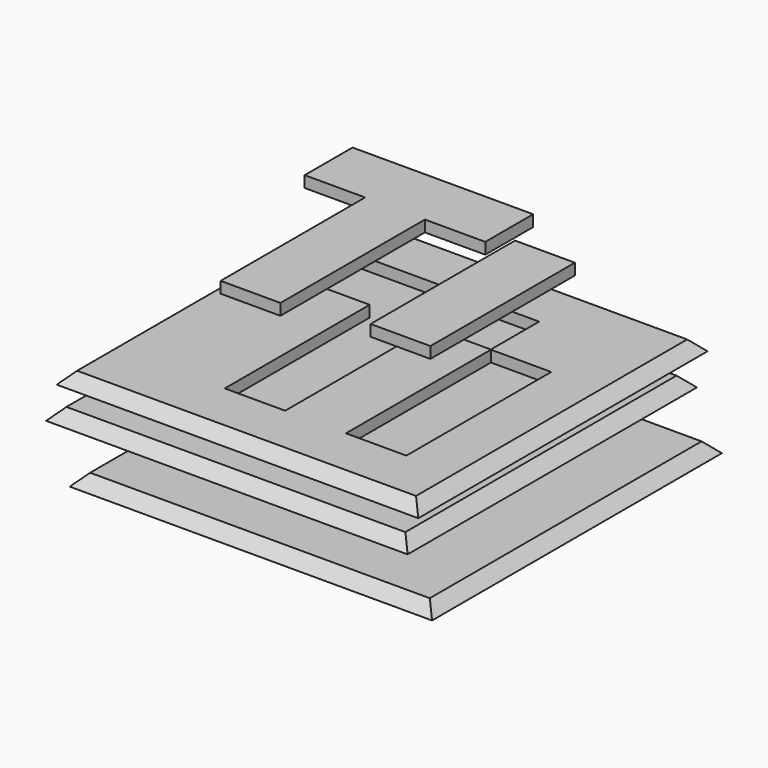
from build123d import *

# Parameters (mm, degrees)
F0_W      = 192
F0_H      = 192
F1_DEPTH  = 6
F2_SIZE   = 5.99999
F4_W      = 191.6
F4_H      = 191.6
F5_DEPTH  = 6
F6_SIZE   = 5.99999
F8_W      = 191.6
F8_H      = 191.6
F9_DEPTH  = 6
F10_SIZE  = 5.99999
F11_W     = 32
F11_H     = 96
F12_DEPTH = 25
F13_W     = 32
F13_H     = 96
F14_DEPTH = 62.001
F16_W     = 31.7
F16_H     = 95.7
F17_DEPTH = 6


# Not quite as in the source:
# - a fillet or chamfer is up to 0.001 mm smaller than in the source, because OpenCascade refuses the exact size


with BuildPart() as f1:
    # F0 (on Top) → F1 (new body)
    with BuildSketch(Plane.XY):
        with Locations((-14.7799842507, -12.9291996509)):
            Rectangle(F0_W, F0_H)
    extrude(amount=F1_DEPTH)

    # F2 (size 6 in the source; OpenCascade refuses exactly that, so slightly less here)
    f2_edges = [f1.edges().sort_by_distance(p)[0] for p in [
        (-14.779984, 83.0708, 6),
        (-110.779984, -12.9292, 6),
        (-14.779984, -108.9292, 6),
        (81.220016, -12.9292, 6),
    ]]
    chamfer(f2_edges, length=F2_SIZE)


with BuildPart() as f5:
    # F4 (on offset) → F5 (new body)
    with BuildSketch(Plane.XY.offset(31)):
        with Locations((-22.2688633949, -19.6866440775)):
            Rectangle(F4_W, F4_H)
    extrude(amount=F5_DEPTH)

    # F6 (size 6 in the source; OpenCascade refuses exactly that, so slightly less here)
    f6_edges = [f5.edges().sort_by_distance(p)[0] for p in [
        (-22.268863, 76.113356, 37),
        (-118.068863, -19.686644, 37),
        (-22.268863, -115.486644, 37),
        (73.531137, -19.686644, 37),
    ]]
    chamfer(f6_edges, length=F6_SIZE)


with BuildPart() as f9:
    # F8 (on offset) → F9 (new body)
    with BuildSketch(Plane.XY.offset(56)):
        with Locations((-9.0808942914, -29.1196251102)):
            Rectangle(F8_W, F8_H)
    extrude(amount=F9_DEPTH)

    # F10 (size 6 in the source; OpenCascade refuses exactly that, so slightly less here)
    f10_edges = [f9.edges().sort_by_distance(p)[0] for p in [
        (86.719106, -29.119625, 62),
        (-9.080894, 66.680375, 62),
        (-104.880894, -29.119625, 62),
        (-9.080894, -124.919625, 62),
    ]]
    chamfer(f10_edges, length=F10_SIZE)

    # F11 (on face) → F12 (cut)
    with BuildSketch(Plane.XY.offset(62)):
        Polygon((22.9191057086, 34.8803748898), (-73.0808942914, 34.8803748898), (-73.0808942914, 2.8803748898), (-41.2808942914, 2.8803748898), (-9.2808942914, 2.8803748898), (22.9191057086, 2.8803748898), align=None)
        with Locations((-25.2808942914, -45.1196251102)):
            Rectangle(F11_W, F11_H)
    extrude(amount=-F12_DEPTH, mode=Mode.SUBTRACT)

    # F13 (on face) → F14 (cut, through all)
    with BuildSketch(Plane.XY.offset(62)):
        with Locations((39.0191057086, -45.2196251102)):
            Rectangle(F13_W, F13_H)
    extrude(amount=-F14_DEPTH, mode=Mode.SUBTRACT)


with BuildPart() as f17:
    # F16 (on offset) → F17 (new body)
    with BuildSketch(Plane.XY.offset(81)):
        Polygon((-9.1325868409, 70.9719068067), (-104.8325868409, 70.9719068067), (-104.8325868409, 39.2719068067), (-72.8325868409, 39.2719068067), (-41.1325868409, 39.2719068067), (-9.1325868409, 39.2719068067), align=None)
        with Locations((-56.9825868409, -8.5780931933)):
            Rectangle(F16_W, F16_H)
    extrude(amount=F17_DEPTH)


with BuildPart() as f17b:
    # F16 (on offset) → F17, piece 2 (new body)
    with BuildSketch(Plane.XY.offset(81)):
        with Locations((15.6059558275, 0.0141661112)):
            Rectangle(F16_W, F16_H)
    extrude(amount=F17_DEPTH)


solid = Compound([f1.part, f5.part, f9.part, f17.part, f17b.part])
